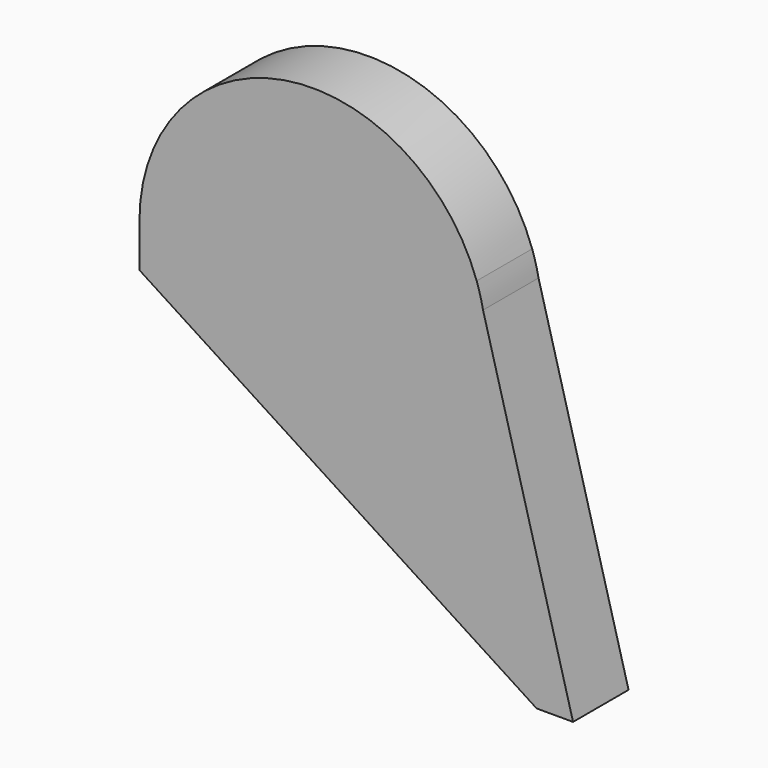
from build123d import *

# Parameters (mm, degrees)
F1_DEPTH = 0.4


# Not quite as in the source:
# - ends of sketch curves that miss each other by under 0.0002 mm in the source are joined


with BuildPart() as f1:
    # F0 (on Front) → F1 (new body)
    with BuildSketch(Plane.XZ):
        with BuildLine():
            ThreePointArc((0.9446077427, 0.3282014815), (-0.166421539, 0.9860547), (-1, 0))
            Line((-1, 0), (-0.9995047651, -0.2500000049))
            Line((-0.9995047651, -0.2500000049), (0.3522404072, -1.1240108766))
            Line((0.3522404072, -1.1240108766), (1.2904977108, -1.73))
            Line((1.2904977108, -1.73), (1.5004977108, -1.73))
            Line((1.5004977108, -1.73), (0.9813866799, 0.1920421425))
            Line((0.9813866799, 0.1920421425), (0.9446077427, 0.3282014815))
        make_face()
        with BuildLine():
            ThreePointArc((0.9813866799, 0.1920421425), (0.9654006787, 0.2607710291), (0.9446077427, 0.3282014815))
            Line((0.9446077427, 0.3282014815), (0.9813866799, 0.1920421425))
        make_face()
    extrude(amount=F1_DEPTH)


solid = f1.part
